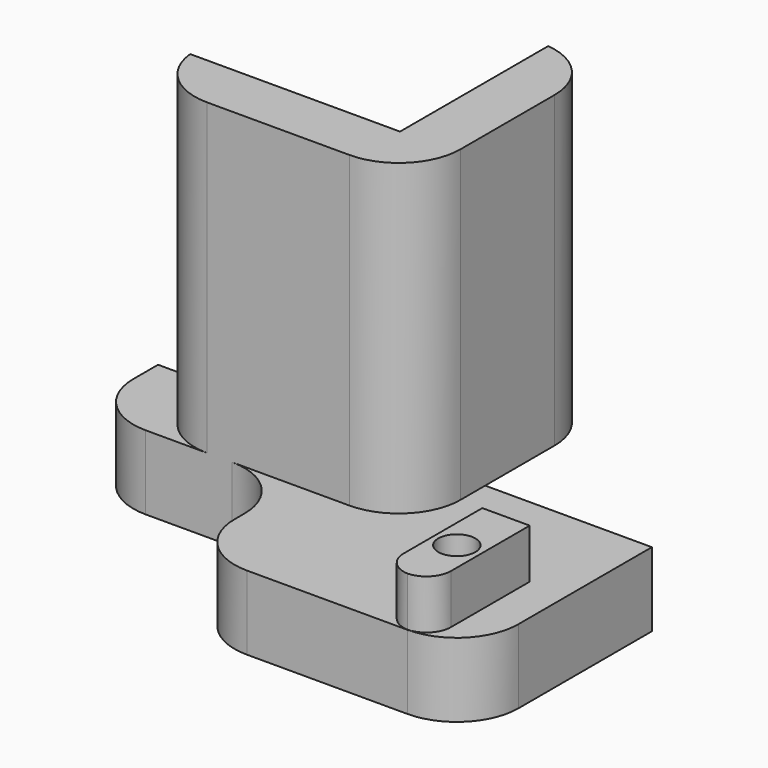
from build123d import *

# Parameters (mm, degrees)
F0_W          = 23
F0_H          = 6
F1_DEPTH      = 11
F2_W          = 3.8415808491
F2_H          = 9.9605580419
F2_R          = 1.5
F3_DEPTH      = 4
F4_DEPTH      = 6
F5_T1_DEPTH   = 9
F6_W          = 23
F6_H          = 6
F6_W_2        = 17
F7_DEPTH      = 4.5
F8_W          = 12
F8_H          = 4.5
F8_W_2        = 5
F9_DEPTH      = 25
F11_DEPTH     = 3
F12_W         = 15
F12_H         = 25
F12_W_2       = 4.5
F13_DEPTH     = 4.5
F14_T1_DEPTH  = 6
F14_T3_DEPTH  = 49.8746859277
F14_T5_DEPTH  = 37.5
F14_T7_DEPTH  = 37.4373429638
F14_T9_DEPTH  = 31
F14_T11_DEPTH = 31
F14_T13_DEPTH = 31


# Not quite as in the source:
# - a fillet or chamfer that OpenCascade refuses, or shapes differently, is made with other operations: its cross-section is extruded or revolved along the edge and cut away or added


with BuildPart() as f1:
    # F0 (on Front) → F1 (new body)
    with BuildSketch(Plane.XZ):
        Rectangle(F0_W, F0_H)
    extrude(amount=-F1_DEPTH)

    # F2 (on face) → F3 (join)
    with BuildSketch(Plane.XY.offset(3)):
        with Locations((6.5, 5)):
            Rectangle(F2_W, F2_H)
        with Locations((6.5, 5)):
            Circle(F2_R, mode=Mode.SUBTRACT)
    extrude(amount=F3_DEPTH)

    # F4 (cut): a face of the model
    f4_faces = [f1.faces().sort_by_distance(p)[0] for p in [
        (6.5, 5, 3),
    ]]
    extrude(f4_faces, amount=-F4_DEPTH, mode=Mode.SUBTRACT)

    # F5: fillet of radius 2 on 2 edges, made by hand

    # F5_s2 → F5_t1 (cut)
    with BuildSketch(Plane.XY.offset(3)):
        with BuildLine():
            ThreePointArc((6.4207904246, 0.019720979), (7.8350039869, 0.6055074167), (8.4207904246, 2.019720979))
            Line((8.4207904246, 2.019720979), (8.4207904246, 0.019720979))
            Line((8.4207904246, 0.019720979), (6.4207904246, 0.019720979))
        make_face()
        with BuildLine():
            ThreePointArc((4.5792095754, 2.019720979), (5.1649960131, 0.6055074167), (6.5792095754, 0.019720979))
            Line((6.5792095754, 0.019720979), (4.5792095754, 0.019720979))
            Line((4.5792095754, 0.019720979), (4.5792095754, 2.019720979))
        make_face()
    extrude(amount=F5_T1_DEPTH, mode=Mode.SUBTRACT)

    # F6 (on face) → F7 (join)
    with BuildSketch(Plane(origin=(0, 11, 0), x_dir=(-1, 0, 0), z_dir=(0, 1, 0))):
        Rectangle(F6_W, F6_H)
        with Locations((20, 0)):
            Rectangle(F6_W_2, F6_H)
    extrude(amount=F7_DEPTH)

    # F8 (on face) → F9 (join)
    with BuildSketch(Plane.XY.offset(3)):
        with Locations((-17.5, 13.25)):
            Rectangle(F8_W, F8_H)
        with Locations((-9, 13.25)):
            Rectangle(F8_W_2, F8_H)
    extrude(amount=F9_DEPTH)

    # F10 (on face) → F11 (join)
    with BuildSketch(Plane(origin=(0, 15.5, 0), x_dir=(-1, 0, 0), z_dir=(0, 1, 0))):
        Polygon((6.5, 3), (-11.5, 3), (-11.5, -3), (28.5, -3), (28.5, 3), (23.5, 3), align=None)
    extrude(amount=F11_DEPTH)

    # F12 (on face) → F13 (join)
    with BuildSketch(Plane.YZ.offset(-6.5)):
        with Locations((23, 15.5)):
            Rectangle(F12_W, F12_H)
        with Locations((13.25, 15.5)):
            Rectangle(F12_W_2, F12_H)
    extrude(amount=F13_DEPTH)

    # F14: fillet of radius 5 on 7 edges, made by hand

    # F14_s2 → F14_t1 (join)
    with BuildSketch(Plane.XY.offset(-3)):
        with BuildLine():
            ThreePointArc((-16.5, 11), (-12.9644660941, 9.5355339059), (-11.5, 6))
            Line((-11.5, 6), (-11.5, 11))
            Line((-11.5, 11), (-16.5, 11))
        make_face()
    extrude(amount=F14_T1_DEPTH)

    # F14_s4 → F14_t3 (cut)
    with BuildSketch(Plane.XY.offset(-9.4373429638)):
        with BuildLine():
            ThreePointArc((-2, 25.5250628145), (-3.2919007565, 28.8791647807), (-6.5, 30.5))
            Line((-6.5, 30.5), (-2, 30.5))
            Line((-2, 30.5), (-2, 25.5250628145))
        make_face()
    extrude(amount=F14_T3_DEPTH, mode=Mode.SUBTRACT)

    # F14_s6 → F14_t5 (cut)
    with BuildSketch(Plane.XY.offset(3)):
        with BuildLine():
            ThreePointArc((-7, 11), (-3.4644660941, 12.4644660941), (-2, 16))
            Line((-2, 16), (-2, 11))
            Line((-2, 11), (-7, 11))
        make_face()
    extrude(amount=F14_T5_DEPTH, mode=Mode.SUBTRACT)

    # F14_s8 → F14_t7 (cut)
    with BuildSketch(Plane.XY.offset(3)):
        with BuildLine():
            ThreePointArc((-18.5250628145, 11), (-21.8791647807, 12.2919007565), (-23.5, 15.5))
            Line((-23.5, 15.5), (-23.5, 11))
            Line((-23.5, 11), (-18.5250628145, 11))
        make_face()
    extrude(amount=F14_T7_DEPTH, mode=Mode.SUBTRACT)

    # F14_s10 → F14_t9 (cut)
    with BuildSketch(Plane.XY.offset(-15.5)):
        with BuildLine():
            ThreePointArc((11.5, 5), (10.0355339059, 1.4644660941), (6.5, 0))
            Line((6.5, 0), (11.5, 0))
            Line((11.5, 0), (11.5, 5))
        make_face()
    extrude(amount=F14_T9_DEPTH, mode=Mode.SUBTRACT)

    # F14_s12 → F14_t11 (cut)
    with BuildSketch(Plane.XY.offset(-15.5)):
        with BuildLine():
            ThreePointArc((-6.5, 0), (-10.0355339059, 1.4644660941), (-11.5, 5))
            Line((-11.5, 5), (-11.5, 0))
            Line((-11.5, 0), (-6.5, 0))
        make_face()
    extrude(amount=F14_T11_DEPTH, mode=Mode.SUBTRACT)

    # F14_s14 → F14_t13 (cut)
    with BuildSketch(Plane.XY.offset(-15.5)):
        with BuildLine():
            ThreePointArc((-28.5, 16), (-27.0355339059, 12.4644660941), (-23.5, 11))
            Line((-23.5, 11), (-28.5, 11))
            Line((-28.5, 11), (-28.5, 16))
        make_face()
    extrude(amount=F14_T13_DEPTH, mode=Mode.SUBTRACT)


solid = f1.part
